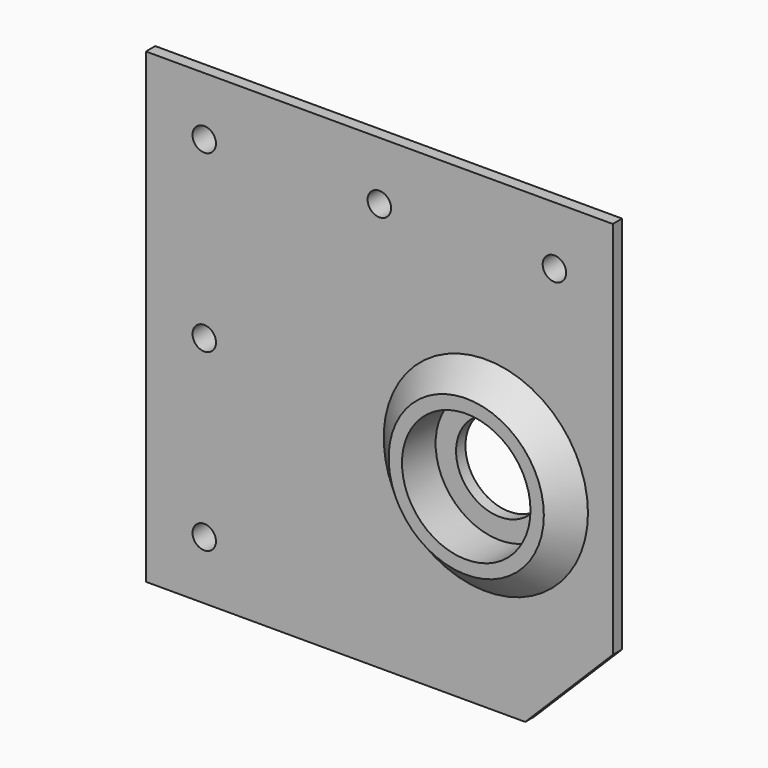
from build123d import *

# Parameters (mm, degrees)
F0_R     = 2.01
F0_R_2   = 7.5
F1_DEPTH = 5
F2_R     = 11.01
F3_DEPTH = 3
F4_R     = 17.5
F4_R_2   = 11.01
F5_DEPTH = 4.2
F6_SIZE  = 4.19999
F7_SIZE  = 3


# Not quite as in the source:
# - a fillet or chamfer is up to 0.001 mm smaller than in the source, because OpenCascade refuses the exact size


with BuildPart() as f1:
    # F0 (on Front) → F1 (new body)
    with BuildSketch(Plane.XZ):
        Polygon((0, 80), (0, 0), (65, 0), (80, 15), (80, 80), align=None)
        with Locations((10, 10)):
            Circle(F0_R, mode=Mode.SUBTRACT)
        with Locations((58.25, 35)):
            Circle(F0_R_2, mode=Mode.SUBTRACT)
        with Locations((10, 40)):
            Circle(F0_R, mode=Mode.SUBTRACT)
        with Locations((10, 70)):
            Circle(F0_R, mode=Mode.SUBTRACT)
        with Locations((40, 70)):
            Circle(F0_R, mode=Mode.SUBTRACT)
        with Locations((70, 70)):
            Circle(F0_R, mode=Mode.SUBTRACT)
    extrude(amount=F1_DEPTH)

    # F2 (on face) → F3 (cut)
    with BuildSketch(Plane.XZ.offset(5)):
        with Locations((58.25, 35)):
            Circle(F2_R)
    extrude(amount=-F3_DEPTH, mode=Mode.SUBTRACT)

    # F4 (on face) → F5 (join)
    with BuildSketch(Plane.XZ.offset(5)):
        with Locations((58.25, 35)):
            Circle(F4_R)
        with Locations((58.25, 35)):
            Circle(F4_R_2, mode=Mode.SUBTRACT)
    extrude(amount=F5_DEPTH)

    # F6 (size 4.2 in the source; OpenCascade refuses exactly that, so slightly less here)
    f6_edges = [f1.edges().sort_by_distance(p)[0] for p in [
        (40.75, -9.2, 35),
    ]]
    chamfer(f6_edges, length=F6_SIZE)

    # F7
    f7_edges = [f1.edges().sort_by_distance(p)[0] for p in [
        (40, 0, 80),
        (80, 0, 47.5),
        (72.5, 0, 7.5),
        (0, 0, 40),
        (32.5, 0, 0),
    ]]
    chamfer(f7_edges, length=F7_SIZE)


with BuildPart() as f8_1:
    # F8: copy of F1
    add(f1.part)


solid = f1.part
